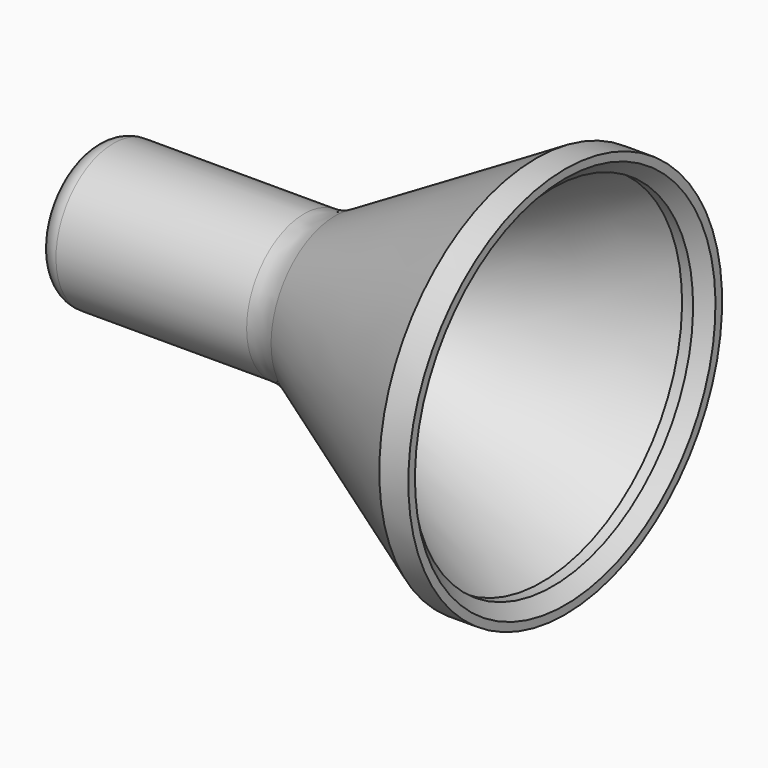
from build123d import *

# Parameters (mm, degrees)
F2_SIZE = 3
F3_R    = 15
F4_R    = 4.99999


# Not quite as in the source:
# - a fillet or chamfer is up to 0.001 mm smaller than in the source, because OpenCascade refuses the exact size


with BuildPart() as f1:
    # F0 (on Front) → F1 (revolve)
    with BuildSketch(Plane.XZ):
        Polygon((55, 17.3), (0, 17.3), (0, 12.3), (56.3397459622, 12.3), (108.3012701892, 42.3), (113.9615242271, 42.3), (113.9615242271, 47.3), (106.9615242271, 47.3), align=None)
    revolve(axis=Axis((19.2044641059, 0, 0), (1, 0, 0)))

    # F2
    f2_edges = [f1.edges().sort_by_distance(p)[0] for p in [
        (113.961524, 0, -42.3),
    ]]
    chamfer(f2_edges, length=F2_SIZE)

    # F3
    f3_edges = [f1.edges().sort_by_distance(p)[0] for p in [
        (55, 0, -17.3),
    ]]
    fillet(f3_edges, radius=F3_R)

    # F4 (radius 5 in the source; OpenCascade refuses exactly that, so slightly less here)
    f4_edges = [f1.edges().sort_by_distance(p)[0] for p in [
        (0, 0, -17.3),
    ]]
    fillet(f4_edges, radius=F4_R)


solid = f1.part
